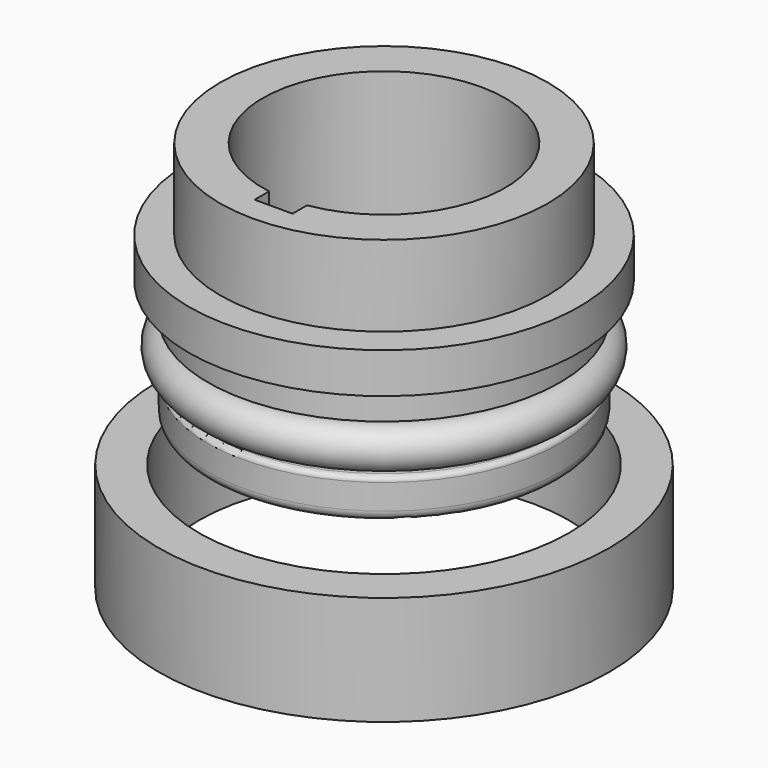
from build123d import *

# Parameters (mm, degrees)
F0_R     = 1
F0_W     = 2
F0_H     = 5.4
F3_DEPTH = 12


# Not quite as in the source:
# - a feature names something its author has since deleted; it is built from what else it names


with BuildPart() as f1:
    # F0 (on Front) → F1 (revolve)
    with BuildSketch(Plane.XZ):
        with BuildLine():
            Line((-9.645, 0), (-8.7, 0))
            Line((-8.7, 0), (-8.7, -1.6))
            Line((-8.7, -1.6), (-7.8666666667, -1.6))
            ThreePointArc((-7.8666666667, -1.6), (-7.5131132761, -1.7464466094), (-7.3666666667, -2.1))
            Line((-7.3666666667, -2.1), (-7.3666666667, -2.8))
            Line((-7.3666666667, -2.8), (-7.3666666667, -3.5))
            ThreePointArc((-7.3666666667, -3.5), (-7.5131132761, -3.8535533906), (-7.8666666667, -4))
            Line((-7.8666666667, -4), (-8.4478927586, -4))
            ThreePointArc((-8.4478927586, -4), (-8.6261594986, -4.0738405014), (-8.7, -4.2521072414))
            Line((-8.7, -4.2521072414), (-8.7, -5.5))
            ThreePointArc((-8.7, -5.5), (-8.5535533906, -5.8535533906), (-8.2, -6))
            Line((-8.2, -6), (-6, -6))
            Line((-6, -6), (-6, 0))
            Line((-6, 0), (-6, 6))
            Line((-6, 6), (-8.1, 6))
            Line((-8.1, 6), (-8.1, 2))
            Line((-8.1, 2), (-9.645, 2))
            Line((-9.645, 2), (-9.645, 0))
        make_face()
    revolve(axis=Axis((0, 0, -0.5250007278), (0, 0, -1)))

    # F2 (on face) → F3 (cut, through all)
    with BuildSketch(Plane.XY.offset(6)):
        with BuildLine():
            Line((-0.9375, -5.926305236), (-0.9375, -6.825))
            Line((-0.9375, -6.825), (0.9375, -6.825))
            Line((0.9375, -6.825), (0.9375, -5.926305236))
            ThreePointArc((0.9375, -5.926305236), (0, -6), (-0.9375, -5.926305236))
        make_face()
    extrude(amount=-F3_DEPTH, mode=Mode.SUBTRACT)


with BuildPart() as f1b:
    # F0 (on Front) → F1, piece 2 (revolve)
    with BuildSketch(Plane.XZ):
        with Locations((-8.3666666667, -2.8)):
            Circle(F0_R)
    revolve(axis=Axis((0, 0, -0.5250007278), (0, 0, -1)))


with BuildPart() as f1c:
    # F0 (on Front) → F1, piece 3 (revolve)
    with BuildSketch(Plane.XZ):
        with Locations((-10.15, -10.7)):
            Rectangle(F0_W, F0_H)
    revolve(axis=Axis((0, 0, -0.5250007278), (0, 0, -1)))


solid = Compound([f1.part, f1b.part, f1c.part])
